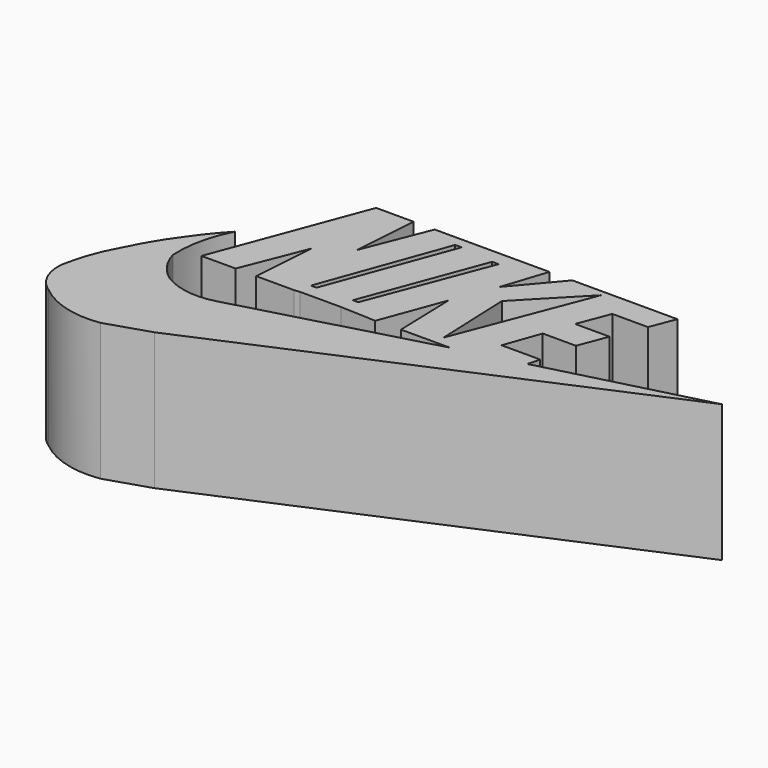
from build123d import *

# Parameters (mm, degrees)
F1_DEPTH = 19.05
F3_DEPTH = 19.05


# Not quite as in the source:
# - a feature names something its author has since deleted; it is built from what else it names


with BuildPart() as f1:
    # F0 (on Top) → F1 (new body)
    with BuildSketch(Plane.XY):
        Polygon((-39.6296493709, 39.737109375), (-44.4920025766, 39.737109375), (-45.0404509902, 38.3060877886), (-51.4150857925, 21.0715923085), (-52.2047057748, 19.1882997751), (-47.2585186362, 19.1882997751), (-46.5040132403, 21.2327073224), (-40.3436794877, 37.7105511725), align=None)
    extrude(amount=F1_DEPTH)



with BuildPart() as f1b:
    # F0 (on Top) → F1, piece 2 (new body)
    with BuildSketch(Plane.XY):
        Polygon((-52.8753772378, 39.737109375), (-58.071937412, 39.737109375), (-65.8153370023, 19.1017910838), (-61.0744804144, 19.1017910838), (-57.5978495181, 27.8723798692), (-58.2299642265, 19.1017910838), (-52.9360063374, 19.1017910838), (-52.2047057748, 21.0715923085), (-45.9454512168, 38.3060877886), (-45.4141758382, 39.737109375), (-49.9411970377, 39.737109375), (-53.4955092069, 30.7705519863), align=None)
    extrude(amount=F1_DEPTH)


with BuildPart() as f1c:
    # F0 (on Top) → F1, piece 3 (new body)
    with BuildSketch(Plane.XY):
        with BuildLine():
            Line((-34.012787044, 39.737109375), (-38.875143975, 39.737109375))
            Line((-38.875143975, 39.737109375), (-39.4490547478, 37.7105511725))
            Line((-39.4490547478, 37.7105511725), (-45.7450146313, 21.2327073224))
            Line((-45.7450146313, 21.2327073224), (-46.5040132403, 19.1882997751))
            Line((-46.5040132403, 19.1882997751), (-41.5926604458, 18.9808556717))
            Line((-41.5926604458, 18.9808556717), (-38.3721441031, 27.6555065066))
            Line((-38.3721441031, 27.6555065066), (-38.1206423044, 19.1044658422))
            Line((-38.1206423044, 19.1044658422), (-31.3301086426, 19.1044658422))
            Line((-31.3301086426, 19.1044658422), (-57.9053983092, 11.8109323084))
            ThreePointArc((-57.9053983092, 11.8109323084), (-61.6554191389, 11.565355508), (-65.1989355683, 12.816936709))
            ThreePointArc((-65.1989355683, 12.816936709), (-67.1816299808, 14.8061054603), (-68.3846175671, 17.3439569771))
            ThreePointArc((-68.3846175671, 17.3439569771), (-68.0426528163, 21.7039427005), (-66.5402710438, 25.8111637086))
            ThreePointArc((-66.5402710438, 25.8111637086), (-68.289988101, 23.8168641952), (-69.8936209083, 21.7033121735))
            ThreePointArc((-69.8936209083, 21.7033121735), (-71.9777744598, 18.6120372362), (-73.74997437, 15.331948176))
            ThreePointArc((-73.74997437, 15.331948176), (-75.226699634, 12.199885885), (-76.2, 8.8767521083))
            ThreePointArc((-76.2, 8.8767521083), (-76.0035829361, 5.2955374253), (-73.74997437, 2.505389275))
            ThreePointArc((-73.74997437, 2.505389275), (-69.4068023904, 0.267420013), (-64.5282641053, 0))
            Line((-64.5282641053, 0), (-58.5760697722, 1.9185534911))
            Line((-58.5760697722, 1.9185534911), (0, 27.1525029093))
            Line((0, 27.1525029093), (-22.3599020392, 21.367976442))
            Line((-22.3599020392, 21.367976442), (-21.9407342374, 23.0446513742))
            Line((-21.9407342374, 23.0446513742), (-27.3060910404, 23.0446513742))
            Line((-27.3060910404, 23.0446513742), (-25.5455821753, 27.9908403754))
            Line((-25.5455821753, 27.9908403754), (-20.9347270429, 27.9908403754))
            Line((-20.9347270429, 27.9908403754), (-19.4257199764, 31.9310240448))
            Line((-19.4257199764, 31.9310240448), (-24.2042429745, 31.9310240448))
            Line((-24.2042429745, 31.9310240448), (-22.5275680423, 36.2903773785))
            Line((-22.5275680423, 36.2903773785), (-17.5813790411, 36.2903773785))
            Line((-17.5813790411, 36.2903773785), (-16.2400398403, 39.737109375))
            Line((-16.2400398403, 39.737109375), (-30.827106908, 39.737109375))
            Line((-30.827106908, 39.737109375), (-36.0247977078, 33.607698977))
            Line((-36.0247977078, 33.607698977), (-34.012787044, 39.737109375))
        make_face()
        Polygon((-26.2162536383, 38.9730595052), (-33.3421193063, 20.5296389759), (-33.7612889707, 31.1765223742), align=None, mode=Mode.SUBTRACT)
    extrude(amount=F1_DEPTH)


with BuildPart() as f1_1:
    add(f1.part)

    add(f1b.part)  # F3 merges F1b

    add(f1c.part)  # F3 merges F1c
    # F2 (on Top) → F3 (join, through all)
    with BuildSketch(Plane.XY):
        Polygon((-39.4490547478, 37.7105511725), (-38.875143975, 39.737109375), (-39.6296493709, 39.737109375), (-40.3436794877, 37.7105511725), align=None)
        Polygon((-46.5040132403, 19.1882997751), (-45.7450146313, 21.2327073224), (-46.5040132403, 21.2327073224), (-47.2585186362, 19.1882997751), align=None)
        Polygon((-52.2047057748, 19.1882997751), (-51.4150857925, 21.0715923085), (-52.2047057748, 21.0715923085), (-52.9360063374, 19.1017910838), align=None)
        Polygon((-45.0404509902, 38.3060877886), (-44.4920025766, 39.737109375), (-45.4141758382, 39.737109375), (-45.9454512168, 38.3060877886), align=None)
    extrude(amount=F3_DEPTH)


solid = f1_1.part
